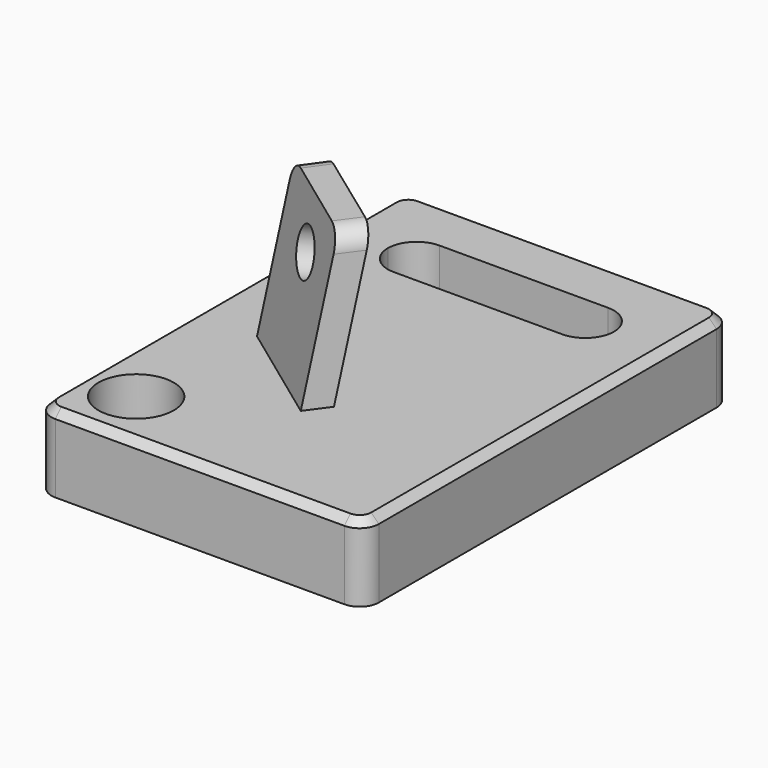
from build123d import *

# Parameters (mm, degrees)
F0_W        = 216.7427750782
F0_H        = 304.8
F0_R        = 24.9340536108
F0_W_2      = 149.6857404709
F0_H_2      = 37.9712283611
F1_DEPTH    = 50.8
F2_T1_DEPTH = 50.8
F3_R        = 12.7
F4_SIZE     = 5.08
F6_DEPTH    = 101.6
F6_FACE1_W  = 86.0803631253
F6_FACE1_H  = 101.6
F9_DEPTH    = 101.6
F10_R       = 12.7
F11_R       = 14.8705082973
F12_DEPTH   = 25.4


# Not quite as in the source:
# - a fillet or chamfer that OpenCascade refuses, or shapes differently, is made with other operations: its cross-section is extruded or revolved along the edge and cut away or added


with BuildPart() as f1:
    # F0 (on Top) → F1 (new body)
    with BuildSketch(Plane.XY):
        Rectangle(F0_W, F0_H)
        with Locations((-72.7102532983, -114.1952574253)):
            Circle(F0_R, mode=Mode.SUBTRACT)
        with Locations((0, 96.7190787196)):
            Rectangle(F0_W_2, F0_H_2, mode=Mode.SUBTRACT)
    extrude(amount=F1_DEPTH)

    # F2: fillet of radius 19.05 on 4 edges, made by hand

    # F2_s2 → F2_t1 (join)
    with BuildSketch(Plane.XY):
        with BuildLine():
            ThreePointArc((-74.8428702354, 96.6546929002), (-69.263254417, 110.1250770818), (-55.7928702354, 115.7046929002))
            Line((-55.7928702354, 115.7046929002), (-74.8428702354, 115.7046929002))
            Line((-74.8428702354, 115.7046929002), (-74.8428702354, 96.6546929002))
        make_face()
        with BuildLine():
            ThreePointArc((-55.7928702354, 77.7334645391), (-69.263254417, 83.3130803574), (-74.8428702354, 96.7834645391))
            Line((-74.8428702354, 96.7834645391), (-74.8428702354, 77.7334645391))
            Line((-74.8428702354, 77.7334645391), (-55.7928702354, 77.7334645391))
        make_face()
        with BuildLine():
            ThreePointArc((74.8428702354, 96.7834645391), (69.263254417, 83.3130803574), (55.7928702354, 77.7334645391))
            Line((55.7928702354, 77.7334645391), (74.8428702354, 77.7334645391))
            Line((74.8428702354, 77.7334645391), (74.8428702354, 96.7834645391))
        make_face()
        with BuildLine():
            ThreePointArc((74.8428702354, 96.6546929002), (69.263254417, 110.1250770818), (55.7928702354, 115.7046929002))
            Line((55.7928702354, 115.7046929002), (74.8428702354, 115.7046929002))
            Line((74.8428702354, 115.7046929002), (74.8428702354, 96.6546929002))
        make_face()
    extrude(amount=F2_T1_DEPTH)

    # F3
    f3_edges = [f1.edges().sort_by_distance(p)[0] for p in [
        (108.371388, 152.4, 25.4),
        (-108.371388, 152.4, 25.4),
        (-108.371388, -152.4, 25.4),
        (108.371388, -152.4, 25.4),
    ]]
    fillet(f3_edges, radius=F3_R)

    # F4
    f4_edges = [f1.edges().sort_by_distance(p)[0] for p in [
        (0, -152.4, 50.8),
        (108.371388, 0, 50.8),
        (104.651644, -148.680256, 50.8),
        (-108.371388, 0, 50.8),
        (-104.651644, -148.680256, 50.8),
        (-104.651644, 148.680256, 50.8),
        (0, 152.4, 50.8),
        (104.651644, 148.680256, 50.8),
    ]]
    chamfer(f4_edges, length=F4_SIZE)

    # F5 (on face) → F6 (join)
    with BuildSketch(Plane.XY.offset(50.8)):
        Polygon((26.1903759085, -43.1183193231), (-44.0938870282, 7.8987490062), (-88.495139861, -54.1171146365), (-18.5043358385, -104.2281540196), align=None)
    extrude(amount=F6_DEPTH)

    # F7 (on face) + F6_face1 (on face) → F9 (cut)
    with BuildSketch(Plane(origin=(37.6086943592, -27.5063704871, 0), x_dir=(0.590339639, 0.8071549484, 0), z_dir=(0.8071549484, -0.590339639, 0))):
        Polygon((-57.197030481, 50.8), (-37.1219477484, 152.4), (-95.0521132136, 152.4), (-95.0521132136, 50.8), align=None)
        Polygon((-19.3419477484, 50.8), (-19.3419477484, 152.4), (-39.417030481, 50.8), align=None)
    with BuildSketch(Plane(origin=(-53.4997378497, -79.172634328, 101.6), x_dir=(0.8130867655, -0.5821425185, 0), z_dir=(-0.5821425185, -0.8130867655, 0))):
        Rectangle(F6_FACE1_W, F6_FACE1_H)
    extrude(amount=-F9_DEPTH, dir=(0.8071549484, -0.590339639, 0), mode=Mode.SUBTRACT)

    # F10 (call 1 of 2: OpenCascade refuses the feature's edges together)
    f10_edges = [f1.edges().sort_by_distance(p)[0] for p in [
        (20.942257, -50.293927, 152.4),
    ]]
    fillet(f10_edges, radius=F10_R)

    # F10#2 (call 2 of 2)
    f10_2_edges = [f1.edges().sort_by_distance(p)[0] for p in [
        (-49.178316, 0.797255, 152.4),
    ]]
    fillet(f10_2_edges, radius=F10_R)

    # F11 (on face) → F12 (cut)
    with BuildSketch(Plane(origin=(-38.199850732, -52.2295921019, 12.7856660343), x_dir=(0.8152262825, -0.5625326873, 0.1377065143), z_dir=(-0.5791425631, -0.7918454983, 0.1938416841))):
        with Locations((20.26450634, 108.0148071051)):
            Circle(F11_R)
    extrude(amount=-F12_DEPTH, mode=Mode.SUBTRACT)


solid = f1.part
